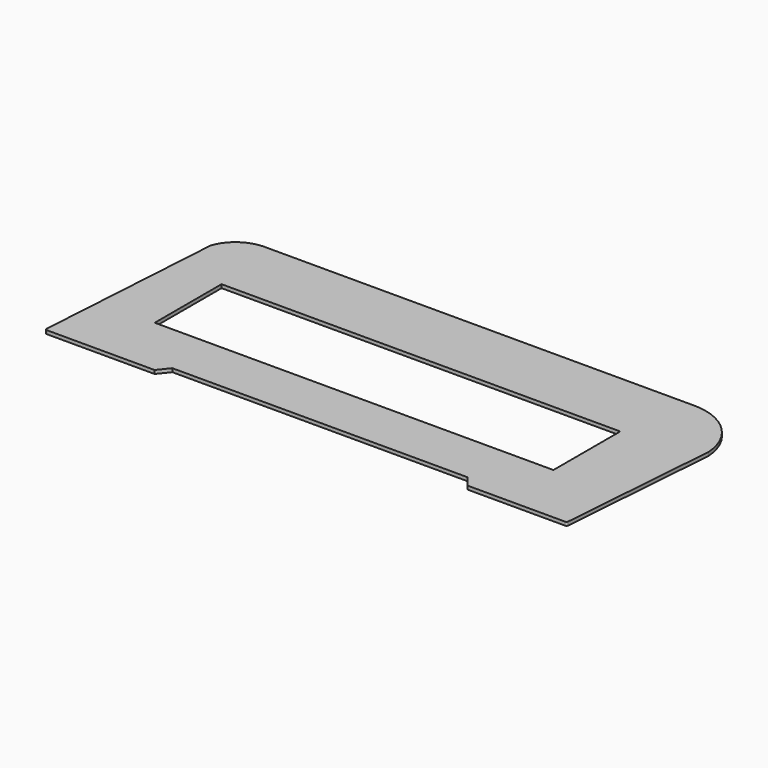
from build123d import *

# Parameters (mm, degrees)
F0_W     = 57.3139749467
F0_H     = 12.0063517243
F1_DEPTH = 0.508


# Not quite as in the source:
# - ends of sketch curves that miss each other by under 0.0002 mm in the source are joined


with BuildPart() as f1:
    # F0 (on Top) → F1 (new body)
    with BuildSketch(Plane.XY):
        with BuildLine():
            Line((-36.7499960837, 12.0419642886), (-38.4861308, -15.2827228))
            ThreePointArc((-38.4861308, -15.2827228), (-38.4148753009, -15.4677583266), (-38.2323086, -15.5451301886))
            Line((-38.2323086, -15.5451301886), (-22.7499926, -15.545054))
            Line((-22.7499926, -15.545054), (-21.4799926, -13.9580366))
            Line((-21.4799926, -13.9580366), (20.9799936, -13.9580366))
            Line((20.9799936, -13.9580366), (22.2499936, -15.545054))
            Line((22.2499936, -15.545054), (36.2593128, -15.545054))
            ThreePointArc((36.2593128, -15.545054), (36.4352434048, -15.4742599559), (36.5131044113, -15.3013407897))
            Line((36.5131044113, -15.3013407897), (38.2500089611, 7.7244699848))
            ThreePointArc((38.2500089611, 7.7244699848), (35.5514966121, 13.3615420014), (29.6945050156, 15.5419546358))
            Line((29.6945050156, 15.5419546358), (-31.9416938, 15.5419806))
            ThreePointArc((-31.9416938, 15.5419806), (-34.897631264, 14.5500112443), (-36.7499960837, 12.0419642886))
        make_face()
        with Locations((-1.2608356774, -0.5606063642)):
            Rectangle(F0_W, F0_H, mode=Mode.SUBTRACT)
    extrude(amount=F1_DEPTH)


solid = f1.part
